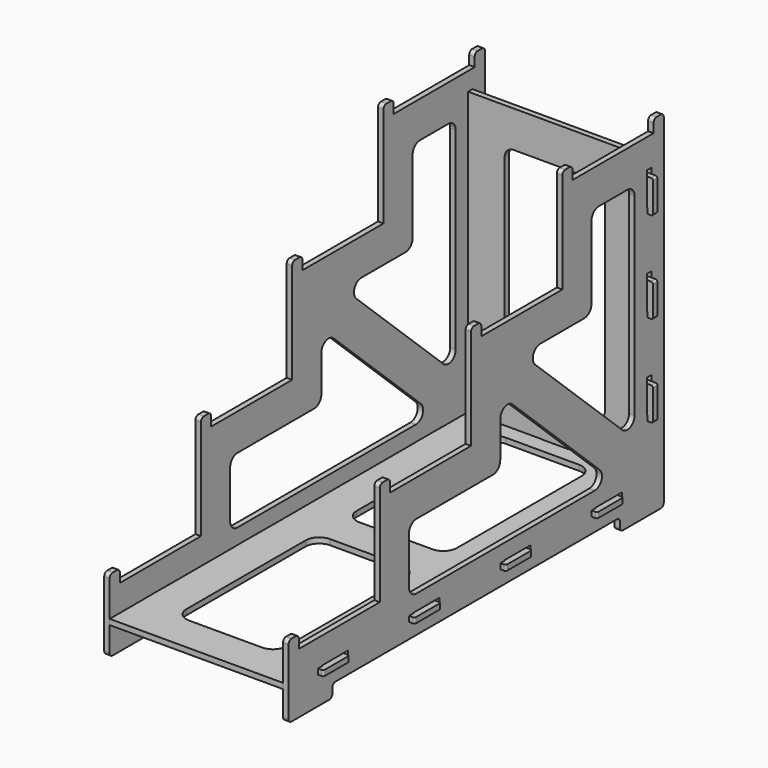
from build123d import *

# Parameters (mm, degrees)
F2_W      = 18
F2_H      = 3.1
F2_W_2    = 3.3
F2_H_2    = 18
F3_DEPTH  = 3
F6_W      = 15
F6_H      = 3.3
F7_DEPTH  = 1.5
F10_DEPTH = 1.5


with BuildPart() as f3:
    # F2 (on offset) → F3 (new body)
    with BuildSketch(Plane.YZ.offset(47.5)):
        with BuildLine():
            Line((-128.5, 38), (-128.5, 2))
            ThreePointArc((-128.5, 2), (-127.9142135624, 0.5857864376), (-126.5, 0))
            Line((-126.5, 0), (-100.5, 0))
            ThreePointArc((-100.5, 0), (-99.0857864376, 0.5857864376), (-98.5, 2))
            Line((-98.5, 2), (-98.5, 5))
            ThreePointArc((-98.5, 5), (-97.9142135624, 6.4142135624), (-96.5, 7))
            Line((-96.5, 7), (96.5, 7))
            ThreePointArc((96.5, 7), (97.9142135624, 6.4142135624), (98.5, 5))
            Line((98.5, 5), (98.5, 2))
            ThreePointArc((98.5, 2), (99.0857864376, 0.5857864376), (100.5, 0))
            Line((100.5, 0), (126.5, 0))
            ThreePointArc((126.5, 0), (127.9142135624, 0.5857864376), (128.5, 2))
            Line((128.5, 2), (128.5, 188))
            ThreePointArc((128.5, 188), (127.9142135624, 189.4142135624), (126.5, 190))
            Line((126.5, 190), (123.5, 190))
            ThreePointArc((123.5, 190), (122.0857864376, 189.4142135624), (121.5, 188))
            Line((121.5, 188), (121.5, 183))
            Line((121.5, 183), (66, 183))
            Line((66, 183), (66, 188))
            ThreePointArc((66, 188), (65.4142135624, 189.4142135624), (64, 190))
            Line((64, 190), (61, 190))
            ThreePointArc((61, 190), (59.5857864376, 189.4142135624), (59, 188))
            Line((59, 188), (59, 133))
            Line((59, 133), (3.5, 133))
            Line((3.5, 133), (3.5, 138))
            ThreePointArc((3.5, 138), (2.9142135624, 139.4142135624), (1.5, 140))
            Line((1.5, 140), (-1.5, 140))
            ThreePointArc((-1.5, 140), (-2.9142135624, 139.4142135624), (-3.5, 138))
            Line((-3.5, 138), (-3.5, 83))
            Line((-3.5, 83), (-59, 83))
            Line((-59, 83), (-59, 88))
            ThreePointArc((-59, 88), (-59.5857864376, 89.4142135624), (-61, 90))
            Line((-61, 90), (-64, 90))
            ThreePointArc((-64, 90), (-65.4142135624, 89.4142135624), (-66, 88))
            Line((-66, 88), (-66, 33))
            Line((-66, 33), (-121.5, 33))
            Line((-121.5, 33), (-121.5, 38))
            ThreePointArc((-121.5, 38), (-122.0857864376, 39.4142135624), (-123.5, 40))
            Line((-123.5, 40), (-126.5, 40))
            ThreePointArc((-126.5, 40), (-127.9142135624, 39.4142135624), (-128.5, 38))
        make_face()
        with Locations((-96.75, 17)):
            Rectangle(F2_W, F2_H, mode=Mode.SUBTRACT)
        with Locations((-34.25, 17)):
            Rectangle(F2_W, F2_H, mode=Mode.SUBTRACT)
        with Locations((28.25, 17)):
            Rectangle(F2_W, F2_H, mode=Mode.SUBTRACT)
        with Locations((90.75, 17)):
            Rectangle(F2_W, F2_H, mode=Mode.SUBTRACT)
        with BuildLine():
            ThreePointArc((-41, 27), (-44.5355339059, 28.4644660941), (-46, 32))
            Line((-46, 32), (-46, 58))
            ThreePointArc((-46, 58), (-44.5355339059, 61.5355339059), (-41, 63))
            Line((-41, 63), (11.5, 63))
            ThreePointArc((11.5, 63), (15.0355339059, 64.4644660941), (16.5, 68))
            Line((16.5, 68), (16.5, 87.792963272))
            ThreePointArc((16.5, 87.792963272), (19.5090325155, 92.3794704917), (24.9144193903, 91.4455979687))
            Line((24.9144193903, 91.4455979687), (84.5999149837, 35.6526346966))
            ThreePointArc((84.5999149837, 35.6526346966), (85.8364725597, 30.1646762524), (81.1854955934, 27))
            Line((81.1854955934, 27), (-41, 27))
        make_face(mode=Mode.SUBTRACT)
        with Locations((118.5, 58)):
            Rectangle(F2_W_2, F2_H_2, mode=Mode.SUBTRACT)
        with BuildLine():
            ThreePointArc((40.4000850163, 104.3473653034), (39.1635274403, 109.8353237476), (43.8145044066, 113))
            Line((43.8145044066, 113), (74, 113))
            ThreePointArc((74, 113), (77.5355339059, 114.4644660941), (79, 118))
            Line((79, 118), (79, 158))
            ThreePointArc((79, 158), (80.4644660941, 161.5355339059), (84, 163))
            Line((84, 163), (103.5, 163))
            ThreePointArc((103.5, 163), (107.0355339059, 161.5355339059), (108.5, 158))
            Line((108.5, 158), (108.5, 52.207036728))
            ThreePointArc((108.5, 52.207036728), (105.4909674845, 47.6205295083), (100.0855806097, 48.5544020313))
            Line((100.0855806097, 48.5544020313), (40.4000850163, 104.3473653034))
        make_face(mode=Mode.SUBTRACT)
        with Locations((118.5, 108)):
            Rectangle(F2_W_2, F2_H_2, mode=Mode.SUBTRACT)
        with Locations((118.5, 158)):
            Rectangle(F2_W_2, F2_H_2, mode=Mode.SUBTRACT)
    extrude(amount=F3_DEPTH)


with BuildPart() as f4_1:
    # F4: instance of F3
    add(f3.part.mirror(Plane.YZ))


with BuildPart() as f7:
    # F6 (on plane+point) → F7 (new body, symmetric)
    with BuildSketch(Plane.XY.offset(17)):
        with BuildLine():
            Line((47.5, 128.5), (0, 128.5))
            Line((0, 128.5), (-47.5, 128.5))
            Line((-47.5, 128.5), (-47.5, 96.75))
            Line((-47.5, 96.75), (-52.8, 96.75))
            ThreePointArc((-52.8, 96.75), (-53.5071067812, 96.4571067812), (-53.8, 95.75))
            Line((-53.8, 95.75), (-53.8, 79.75))
            ThreePointArc((-53.8, 79.75), (-53.5071067812, 79.0428932188), (-52.8, 78.75))
            Line((-52.8, 78.75), (-50.8, 78.75))
            Line((-50.8, 78.75), (-50.8, 81.75))
            Line((-50.8, 81.75), (-47.5, 81.75))
            Line((-47.5, 81.75), (-47.5, 34.25))
            Line((-47.5, 34.25), (-52.8, 34.25))
            ThreePointArc((-52.8, 34.25), (-53.5071067812, 33.9571067812), (-53.8, 33.25))
            Line((-53.8, 33.25), (-53.8, 17.25))
            ThreePointArc((-53.8, 17.25), (-53.5071067812, 16.5428932188), (-52.8, 16.25))
            Line((-52.8, 16.25), (-50.8, 16.25))
            Line((-50.8, 16.25), (-50.8, 19.25))
            Line((-50.8, 19.25), (-47.5, 19.25))
            Line((-47.5, 19.25), (-47.5, -28.25))
            Line((-47.5, -28.25), (-52.8, -28.25))
            ThreePointArc((-52.8, -28.25), (-53.5071067812, -28.5428932188), (-53.8, -29.25))
            Line((-53.8, -29.25), (-53.8, -45.25))
            ThreePointArc((-53.8, -45.25), (-53.5071067812, -45.9571067812), (-52.8, -46.25))
            Line((-52.8, -46.25), (-50.8, -46.25))
            Line((-50.8, -46.25), (-50.8, -43.25))
            Line((-50.8, -43.25), (-47.5, -43.25))
            Line((-47.5, -43.25), (-47.5, -90.75))
            Line((-47.5, -90.75), (-52.8, -90.75))
            ThreePointArc((-52.8, -90.75), (-53.5071067812, -91.0428932188), (-53.8, -91.75))
            Line((-53.8, -91.75), (-53.8, -107.75))
            ThreePointArc((-53.8, -107.75), (-53.5071067812, -108.4571067812), (-52.8, -108.75))
            Line((-52.8, -108.75), (-50.8, -108.75))
            Line((-50.8, -108.75), (-50.8, -105.75))
            Line((-50.8, -105.75), (-47.5, -105.75))
            Line((-47.5, -105.75), (-47.5, -128.5))
            Line((-47.5, -128.5), (0, -128.5))
            Line((0, -128.5), (47.5, -128.5))
            Line((47.5, -128.5), (47.5, -105.75))
            Line((47.5, -105.75), (50.8, -105.75))
            Line((50.8, -105.75), (50.8, -108.75))
            Line((50.8, -108.75), (52.8, -108.75))
            ThreePointArc((52.8, -108.75), (53.5071067812, -108.4571067812), (53.8, -107.75))
            Line((53.8, -107.75), (53.8, -91.75))
            ThreePointArc((53.8, -91.75), (53.5071067812, -91.0428932188), (52.8, -90.75))
            Line((52.8, -90.75), (47.5, -90.75))
            Line((47.5, -90.75), (47.5, -43.25))
            Line((47.5, -43.25), (50.8, -43.25))
            Line((50.8, -43.25), (50.8, -46.25))
            Line((50.8, -46.25), (52.8, -46.25))
            ThreePointArc((52.8, -46.25), (53.5071067812, -45.9571067812), (53.8, -45.25))
            Line((53.8, -45.25), (53.8, -29.25))
            ThreePointArc((53.8, -29.25), (53.5071067812, -28.5428932188), (52.8, -28.25))
            Line((52.8, -28.25), (47.5, -28.25))
            Line((47.5, -28.25), (47.5, 19.25))
            Line((47.5, 19.25), (50.8, 19.25))
            Line((50.8, 19.25), (50.8, 16.25))
            Line((50.8, 16.25), (52.8, 16.25))
            ThreePointArc((52.8, 16.25), (53.5071067812, 16.5428932188), (53.8, 17.25))
            Line((53.8, 17.25), (53.8, 33.25))
            ThreePointArc((53.8, 33.25), (53.5071067812, 33.9571067812), (52.8, 34.25))
            Line((52.8, 34.25), (47.5, 34.25))
            Line((47.5, 34.25), (47.5, 81.75))
            Line((47.5, 81.75), (50.8, 81.75))
            Line((50.8, 81.75), (50.8, 78.75))
            Line((50.8, 78.75), (52.8, 78.75))
            ThreePointArc((52.8, 78.75), (53.5071067812, 79.0428932188), (53.8, 79.75))
            Line((53.8, 79.75), (53.8, 95.75))
            ThreePointArc((53.8, 95.75), (53.5071067812, 96.4571067812), (52.8, 96.75))
            Line((52.8, 96.75), (47.5, 96.75))
            Line((47.5, 96.75), (47.5, 128.5))
        make_face()
        with BuildLine():
            Line((20, -108.5), (-20, -108.5))
            ThreePointArc((-20, -108.5), (-25.3033008589, -106.3033008589), (-27.5, -101))
            Line((-27.5, -101), (-27.5, -19.3664571794))
            ThreePointArc((-27.5, -19.3664571794), (-25.3033008589, -14.0631563205), (-20, -11.8664571794))
            Line((-20, -11.8664571794), (20, -11.8664571794))
            ThreePointArc((20, -11.8664571794), (25.3033008589, -14.0631563205), (27.5, -19.3664571794))
            Line((27.5, -19.3664571794), (27.5, -101))
            ThreePointArc((27.5, -101), (25.3033008589, -106.3033008589), (20, -108.5))
        make_face(mode=Mode.SUBTRACT)
        Polygon((-43.6060604866, 126.5), (-43.1290498776, 126.5), (-44.6994517606, 123.1061732153), (-42.633788428, 123.1061732153), (-42.633788428, 122.7096322221), (-45.1557227779, 122.7096322221), (-45.1557227779, 123.0547390279), align=None, mode=Mode.SUBTRACT)
        with BuildLine():
            Line((-41.2077341031, 122.7096322221), (-41.2077341031, 126.5))
            Line((-41.2077341031, 126.5), (-40.7879647673, 126.5))
            Line((-40.7879647673, 126.5), (-40.7879647673, 123.7988755779))
            add(Edge.make_bspline(
                [(-40.7879647673, 123.7988755779), (-40.7879647673, 123.4612350251), (-40.808704359, 123.1609257374)],
                knots=[0, 0, 0, 1, 1, 1], degree=2))
            add(Edge.make_bspline(
                [(-40.808704359, 123.1609257374), (-40.7547814205, 123.2156782594), (-40.6871703516, 123.2749934917)],
                knots=[0, 0, 0, 1, 1, 1], degree=2))
            add(Edge.make_bspline(
                [(-40.6871703516, 123.2749934917), (-40.6195592827, 123.3343087239), (-40.0703748947, 123.7806247372)],
                knots=[0, 0, 0, 1, 1, 1], degree=2))
            Line((-40.0703748947, 123.7806247372), (-39.842239386, 123.4852929514))
            Line((-39.842239386, 123.4852929514), (-40.8452060403, 122.7096322221))
            Line((-40.8452060403, 122.7096322221), (-41.2077341031, 122.7096322221))
        make_face(mode=Mode.SUBTRACT)
        Polygon((-38.5248605217, 122.7096322221), (-39.0068486326, 122.7096322221), (-38.9031506742, 124.0784452739), (-38.6310472311, 124.0784452739), align=None, mode=Mode.SUBTRACT)
        with BuildLine():
            Line((-35.9340707273, 125.8827897512), (-36.4061038343, 125.8827897512))
            Line((-36.4061038343, 125.8827897512), (-36.4450942667, 125.9425197753))
            add(Edge.make_bspline(
                [(-36.4450942667, 125.9425197753), (-36.3770684059, 126.2021794633), (-36.2501421047, 126.5456271017)],
                knots=[0, 0, 0, 1, 1, 1], degree=2))
            add(Edge.make_bspline(
                [(-36.2501421047, 126.5456271017), (-36.1232158036, 126.8890747402), (-35.9863344984, 127.1844065259)],
                knots=[0, 0, 0, 1, 1, 1], degree=2))
            Line((-35.9863344984, 127.1844065259), (-35.6619672843, 127.1844065259))
            add(Edge.make_bspline(
                [(-35.6619672843, 127.1844065259), (-35.7316523124, 126.9147918339), (-35.8158550547, 126.5182508407)],
                knots=[0, 0, 0, 1, 1, 1], degree=2))
            add(Edge.make_bspline(
                [(-35.8158550547, 126.5182508407), (-35.900057797, 126.1217098475), (-35.9340707273, 125.8827897512)],
                knots=[0, 0, 0, 1, 1, 1], degree=2))
        make_face(mode=Mode.SUBTRACT)
        with BuildLine():
            add(Edge.make_bspline(
                [(-35.0198695255, 124.8590835052), (-35.2438571158, 125.1029811035), (-35.2438571158, 125.49122626)],
                knots=[0, 0, 0, 1, 1, 1], degree=2))
            add(Edge.make_bspline(
                [(-35.2438571158, 125.49122626), (-35.2438571158, 125.9914652117), (-34.8809142611, 126.2718644914)],
                knots=[0, 0, 0, 1, 1, 1], degree=2))
            add(Edge.make_bspline(
                [(-34.8809142611, 126.2718644914), (-34.5179714065, 126.5522637711), (-33.8957836557, 126.5522637711)],
                knots=[0, 0, 0, 1, 1, 1], degree=2))
            add(Edge.make_bspline(
                [(-33.8957836557, 126.5522637711), (-33.2221617175, 126.5522637711), (-32.858804071, 126.3780512008)],
                knots=[0, 0, 0, 1, 1, 1], degree=2))
            Line((-32.858804071, 126.3780512008), (-32.858804071, 125.953304363))
            add(Edge.make_bspline(
                [(-32.858804071, 125.953304363), (-33.0927466653, 126.0511952358), (-33.3673388594, 126.1084365088)],
                knots=[0, 0, 0, 1, 1, 1], degree=2))
            add(Edge.make_bspline(
                [(-33.3673388594, 126.1084365088), (-33.6419310534, 126.1656777819), (-33.9115457454, 126.1656777819)],
                knots=[0, 0, 0, 1, 1, 1], degree=2))
            add(Edge.make_bspline(
                [(-33.9115457454, 126.1656777819), (-34.352054673, 126.1656777819), (-34.5752126796, 125.9985166729)],
                knots=[0, 0, 0, 1, 1, 1], degree=2))
            add(Edge.make_bspline(
                [(-34.5752126796, 125.9985166729), (-34.7983706862, 125.8313555638), (-34.7983706862, 125.5327054434)],
                knots=[0, 0, 0, 1, 1, 1], degree=2))
            add(Edge.make_bspline(
                [(-34.7983706862, 125.5327054434), (-34.7983706862, 125.3360941142), (-34.7191454459, 125.2104121885)],
                knots=[0, 0, 0, 1, 1, 1], degree=2))
            add(Edge.make_bspline(
                [(-34.7191454459, 125.2104121885), (-34.6399202057, 125.0847302628), (-34.4545082559, 124.9781287615)],
                knots=[0, 0, 0, 1, 1, 1], degree=2))
            add(Edge.make_bspline(
                [(-34.4545082559, 124.9781287615), (-34.2690963062, 124.8715272602), (-33.8908061537, 124.7371347061)],
                knots=[0, 0, 0, 1, 1, 1], degree=2))
            add(Edge.make_bspline(
                [(-33.8908061537, 124.7371347061), (-33.3623613574, 124.5479896298), (-33.1354702242, 124.2887447336)],
                knots=[0, 0, 0, 1, 1, 1], degree=2))
            add(Edge.make_bspline(
                [(-33.1354702242, 124.2887447336), (-32.9085790911, 124.0294998375), (-32.9085790911, 123.6122192526)],
                knots=[0, 0, 0, 1, 1, 1], degree=2))
            add(Edge.make_bspline(
                [(-32.9085790911, 123.6122192526), (-32.9085790911, 123.174199076), (-33.2375090154, 122.9149541799)],
                knots=[0, 0, 0, 1, 1, 1], degree=2))
            add(Edge.make_bspline(
                [(-33.2375090154, 122.9149541799), (-33.5664389396, 122.6557092837), (-34.1089866583, 122.6557092837)],
                knots=[0, 0, 0, 1, 1, 1], degree=2))
            add(Edge.make_bspline(
                [(-34.1089866583, 122.6557092837), (-34.673933136, 122.6557092837), (-35.148454994, 122.8631052006)],
                knots=[0, 0, 0, 1, 1, 1], degree=2))
            Line((-35.148454994, 122.8631052006), (-35.0107441051, 123.2463728551))
            add(Edge.make_bspline(
                [(-35.0107441051, 123.2463728551), (-34.5411997492, 123.0497615259), (-34.0982020706, 123.0497615259)],
                knots=[0, 0, 0, 1, 1, 1], degree=2))
            add(Edge.make_bspline(
                [(-34.0982020706, 123.0497615259), (-33.7481177629, 123.0497615259), (-33.5510916418, 123.1999161697)],
                knots=[0, 0, 0, 1, 1, 1], degree=2))
            add(Edge.make_bspline(
                [(-33.5510916418, 123.1999161697), (-33.3540655207, 123.3500708136), (-33.3540655207, 123.6171967546)],
                knots=[0, 0, 0, 1, 1, 1], degree=2))
            add(Edge.make_bspline(
                [(-33.3540655207, 123.6171967546), (-33.3540655207, 123.8138080839), (-33.4266540916, 123.9399048014)],
                knots=[0, 0, 0, 1, 1, 1], degree=2))
            add(Edge.make_bspline(
                [(-33.4266540916, 123.9399048014), (-33.4992426625, 124.0660015189), (-33.6717960654, 124.1709438528)],
                knots=[0, 0, 0, 1, 1, 1], degree=2))
            add(Edge.make_bspline(
                [(-33.6717960654, 124.1709438528), (-33.8443494683, 124.2758861868), (-34.1994112781, 124.402812488)],
                knots=[0, 0, 0, 1, 1, 1], degree=2))
            add(Edge.make_bspline(
                [(-34.1994112781, 124.402812488), (-34.7958819352, 124.6151859069), (-35.0198695255, 124.8590835052)],
                knots=[0, 0, 0, 1, 1, 1], degree=2))
        make_face(mode=Mode.SUBTRACT)
        Polygon((-31.2419455026, 123.3401158096), (-31.2419455026, 124.4492691734), (-32.309619683, 124.4492691734), (-32.309619683, 124.8068197342), (-31.2419455026, 124.8068197342), (-31.2419455026, 125.9118251796), (-30.8810766072, 125.9118251796), (-30.8810766072, 124.8068197342), (-29.8183799288, 124.8068197342), (-29.8183799288, 124.4492691734), (-30.8810766072, 124.4492691734), (-30.8810766072, 123.3401158096), align=None, mode=Mode.SUBTRACT)
        with BuildLine():
            Line((-29.0277866934, 122.7096322221), (-29.0277866934, 126.5))
            Line((-29.0277866934, 126.5), (-28.5250589908, 126.5))
            Line((-28.5250589908, 126.5), (-26.4535885724, 123.3193762179))
            Line((-26.4535885724, 123.3193762179), (-26.4328489808, 123.3193762179))
            add(Edge.make_bspline(
                [(-26.4328489808, 123.3193762179), (-26.4743281641, 123.8793451936), (-26.4743281641, 124.3455712149)],
                knots=[0, 0, 0, 1, 1, 1], degree=2))
            Line((-26.4743281641, 124.3455712149), (-26.4743281641, 126.5))
            Line((-26.4743281641, 126.5), (-26.0670025833, 126.5))
            Line((-26.0670025833, 126.5), (-26.0670025833, 122.7096322221))
            Line((-26.0670025833, 122.7096322221), (-26.5647527839, 122.7096322221))
            Line((-26.5647527839, 122.7096322221), (-28.6312457003, 125.8778122492))
            Line((-28.6312457003, 125.8778122492), (-28.6519852919, 125.8778122492))
            add(Edge.make_bspline(
                [(-28.6519852919, 125.8778122492), (-28.6470077899, 125.8081272211), (-28.6287569493, 125.4281779013)],
                knots=[0, 0, 0, 1, 1, 1], degree=2))
            add(Edge.make_bspline(
                [(-28.6287569493, 125.4281779013), (-28.6105061086, 125.0482285815), (-28.6154836106, 124.8848005989)],
                knots=[0, 0, 0, 1, 1, 1], degree=2))
            Line((-28.6154836106, 124.8848005989), (-28.6154836106, 122.7096322221))
            Line((-28.6154836106, 122.7096322221), (-29.0277866934, 122.7096322221))
        make_face(mode=Mode.SUBTRACT)
        with BuildLine():
            Line((20, 8.1335428206), (-20, 8.1335428206))
            ThreePointArc((-20, 8.1335428206), (-25.3033008589, 10.3302419617), (-27.5, 15.6335428206))
            Line((-27.5, 15.6335428206), (-27.5, 101))
            ThreePointArc((-27.5, 101), (-25.3033008589, 106.3033008589), (-20, 108.5))
            Line((-20, 108.5), (20, 108.5))
            ThreePointArc((20, 108.5), (25.3033008589, 106.3033008589), (27.5, 101))
            Line((27.5, 101), (27.5, 15.6335428206))
            ThreePointArc((27.5, 15.6335428206), (25.3033008589, 10.3302419617), (20, 8.1335428206))
        make_face(mode=Mode.SUBTRACT)
        with Locations((0, 118.5)):
            Rectangle(F6_W, F6_H, mode=Mode.SUBTRACT)
    extrude(amount=F7_DEPTH, both=True)


with BuildPart() as f10:
    # F9 (on plane+point) → F10 (new body, symmetric)
    with BuildSketch(Plane.XZ.offset(-118.5)):
        with BuildLine():
            Line((-6.2454659663, 16.0125314072), (0, 16.0125314072))
            Line((0, 16.0125314072), (6.2454659663, 16.0125314072))
            ThreePointArc((6.2454659663, 16.0125314072), (6.9162863595, 16.2709115585), (7.2404534034, 16.9125314072))
            Line((7.2404534034, 16.9125314072), (7.4, 18.5))
            Line((7.4, 18.5), (47.5, 18.5))
            Line((47.5, 18.5), (47.5, 49))
            Line((47.5, 49), (50.8, 49))
            Line((50.8, 49), (50.8, 46))
            Line((50.8, 46), (52.8, 46))
            ThreePointArc((52.8, 46), (53.5071067812, 46.2928932188), (53.8, 47))
            Line((53.8, 47), (53.8, 63))
            ThreePointArc((53.8, 63), (53.5071067812, 63.7071067812), (52.8, 64))
            Line((52.8, 64), (47.5, 64))
            Line((47.5, 64), (47.5, 99))
            Line((47.5, 99), (50.8, 99))
            Line((50.8, 99), (50.8, 96))
            Line((50.8, 96), (52.8, 96))
            ThreePointArc((52.8, 96), (53.5071067812, 96.2928932188), (53.8, 97))
            Line((53.8, 97), (53.8, 113))
            ThreePointArc((53.8, 113), (53.5071067812, 113.7071067812), (52.8, 114))
            Line((52.8, 114), (47.5, 114))
            Line((47.5, 114), (47.5, 149))
            Line((47.5, 149), (50.8, 149))
            Line((50.8, 149), (50.8, 146))
            Line((50.8, 146), (52.8, 146))
            ThreePointArc((52.8, 146), (53.5071067812, 146.2928932188), (53.8, 147))
            Line((53.8, 147), (53.8, 163))
            ThreePointArc((53.8, 163), (53.5071067812, 163.7071067812), (52.8, 164))
            Line((52.8, 164), (47.5, 164))
            Line((47.5, 164), (47.5, 173))
            Line((47.5, 173), (-47.5, 173))
            Line((-47.5, 173), (-47.5, 164))
            Line((-47.5, 164), (-52.8, 164))
            ThreePointArc((-52.8, 164), (-53.5071067812, 163.7071067812), (-53.8, 163))
            Line((-53.8, 163), (-53.8, 147))
            ThreePointArc((-53.8, 147), (-53.5071067812, 146.2928932188), (-52.8, 146))
            Line((-52.8, 146), (-50.8, 146))
            Line((-50.8, 146), (-50.8, 149))
            Line((-50.8, 149), (-47.5, 149))
            Line((-47.5, 149), (-47.5, 114))
            Line((-47.5, 114), (-52.8, 114))
            ThreePointArc((-52.8, 114), (-53.5071067812, 113.7071067812), (-53.8, 113))
            Line((-53.8, 113), (-53.8, 97))
            ThreePointArc((-53.8, 97), (-53.5071067812, 96.2928932188), (-52.8, 96))
            Line((-52.8, 96), (-50.8, 96))
            Line((-50.8, 96), (-50.8, 99))
            Line((-50.8, 99), (-47.5, 99))
            Line((-47.5, 99), (-47.5, 64))
            Line((-47.5, 64), (-52.8, 64))
            ThreePointArc((-52.8, 64), (-53.5071067812, 63.7071067812), (-53.8, 63))
            Line((-53.8, 63), (-53.8, 47))
            ThreePointArc((-53.8, 47), (-53.5071067812, 46.2928932188), (-52.8, 46))
            Line((-52.8, 46), (-50.8, 46))
            Line((-50.8, 46), (-50.8, 49))
            Line((-50.8, 49), (-47.5, 49))
            Line((-47.5, 49), (-47.5, 18.5))
            Line((-47.5, 18.5), (-7.4, 18.5))
            Line((-7.4, 18.5), (-7.2404534034, 16.9125314072))
            ThreePointArc((-7.2404534034, 16.9125314072), (-6.9162863595, 16.2709115585), (-6.2454659663, 16.0125314072))
        make_face()
        with BuildLine():
            Line((-22.5, 153), (22.5, 153))
            ThreePointArc((22.5, 153), (26.0355339059, 151.5355339059), (27.5, 148))
            Line((27.5, 148), (27.5, 43.5))
            ThreePointArc((27.5, 43.5), (26.0355339059, 39.9644660941), (22.5, 38.5))
            Line((22.5, 38.5), (-22.5, 38.5))
            ThreePointArc((-22.5, 38.5), (-26.0355339059, 39.9644660941), (-27.5, 43.5))
            Line((-27.5, 43.5), (-27.5, 148))
            ThreePointArc((-27.5, 148), (-26.0355339059, 151.5355339059), (-22.5, 153))
        make_face(mode=Mode.SUBTRACT)
    extrude(amount=F10_DEPTH, both=True)


solid = Compound([f3.part, f4_1.part, f7.part, f10.part])
